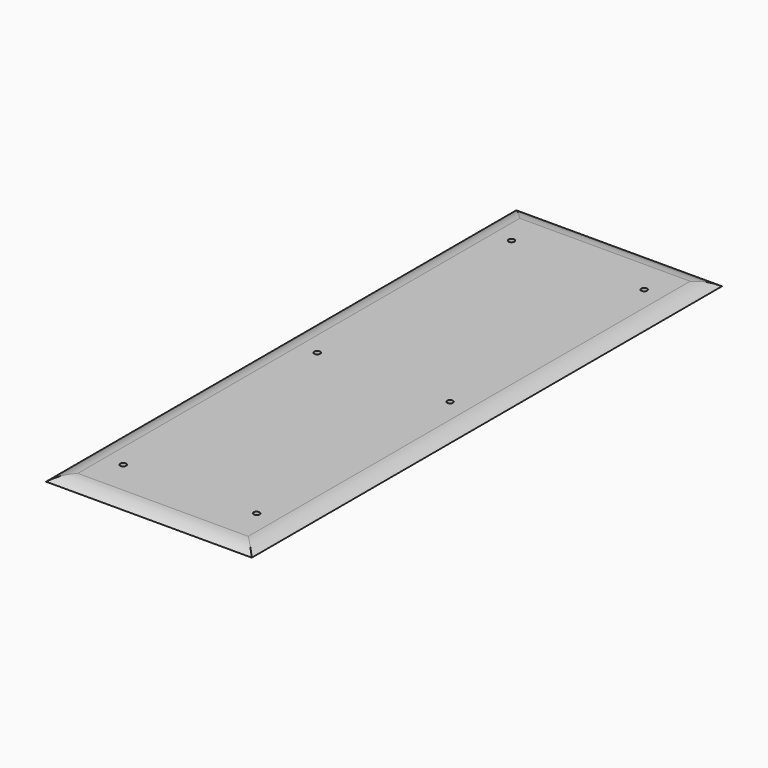
from build123d import *

# Parameters (mm, degrees)
F0_W        = 88.9
F0_H        = 254
F1_DEPTH    = 2.54
F2_T1_DEPTH = 127
F2_T3_DEPTH = 292.1
F5_D        = 2.54
F5_DEPTH    = 5.08
F5_TIP      = 0.7630929862


# Not quite as in the source:
# - a fillet or chamfer that OpenCascade refuses, or shapes differently, is made with other operations: its cross-section is extruded or revolved along the edge and cut away or added


with BuildPart() as f1:
    # F0 (on Top) → F1 (new body)
    with BuildSketch(Plane.XY):
        Rectangle(F0_W, F0_H)
    extrude(amount=F1_DEPTH)

    # F2: fillet of radius 12.7 on 4 edges, made by hand

    # F2_s2 → F2_t1 (cut)
    with BuildSketch(Plane.YZ.offset(-63.5)):
        with BuildLine():
            ThreePointArc((127, 0), (123.3960926284, 1.8882778852), (119.38, 2.54))
            Line((119.38, 2.54), (127, 2.54))
            Line((127, 2.54), (127, 0))
        make_face()
        with BuildLine():
            ThreePointArc((-127, 0), (-123.3960926284, 1.8882778852), (-119.38, 2.54))
            Line((-119.38, 2.54), (-127, 2.54))
            Line((-127, 2.54), (-127, 0))
        make_face()
    extrude(amount=F2_T1_DEPTH, mode=Mode.SUBTRACT)

    # F2_s4 → F2_t3 (cut)
    with BuildSketch(Plane.XZ.offset(-146.05)):
        with BuildLine():
            ThreePointArc((-44.45, 0), (-40.8460926284, 1.8882778852), (-36.83, 2.54))
            Line((-36.83, 2.54), (-44.45, 2.54))
            Line((-44.45, 2.54), (-44.45, 0))
        make_face()
        with BuildLine():
            ThreePointArc((44.45, 0), (40.8460926284, 1.8882778852), (36.83, 2.54))
            Line((36.83, 2.54), (44.45, 2.54))
            Line((44.45, 2.54), (44.45, 0))
        make_face()
    extrude(amount=F2_T3_DEPTH, mode=Mode.SUBTRACT)

    # F5
    with Locations(Plane.XY.offset(2.54)):
        with Locations((-28.8370940834, 104.9257144332), (28.5376422107, 104.9257144332), (28.5376422107, 0), (-28.8370940834, 0), (-28.8370940834, -104.8506721854), (28.5376422107, -104.4920757413)):
            Hole(F5_D / 2, depth=F5_DEPTH)
            with Locations((0, 0, -(F5_DEPTH + F5_TIP / 2))):  # 118° drill point
                Cone(0, F5_D / 2, F5_TIP, mode=Mode.SUBTRACT)


solid = f1.part
